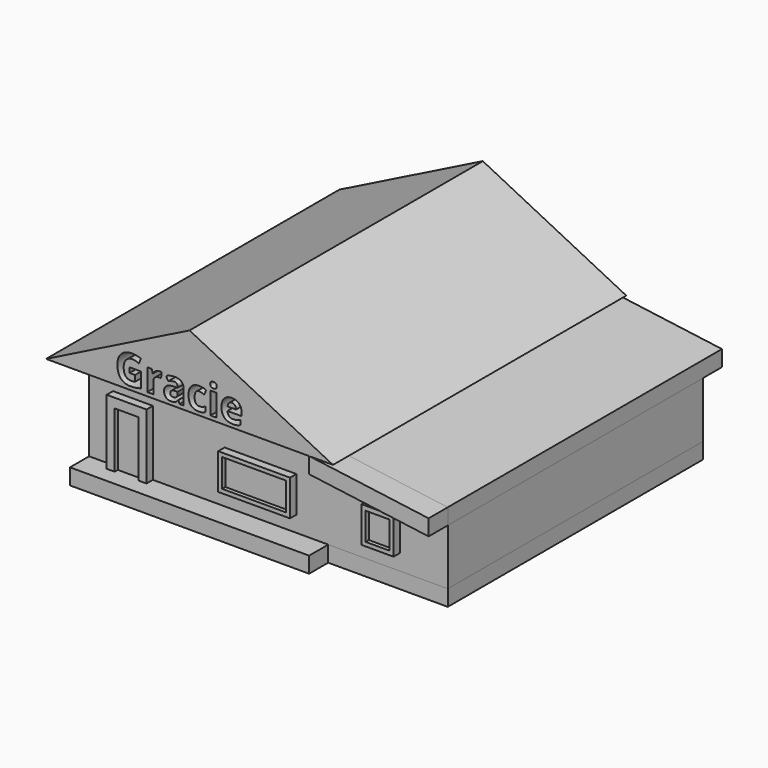
from build123d import *

# Parameters (mm, degrees)
F1_DEPTH      = 914.4
F2_DEPTH      = 13106.4
F3_DEPTH      = 12192
F4_DEPTH      = 914.4
F5_DEPTH      = 12192
F0_W          = 2743.2
F0_H          = 1371.6
F0_W_2        = 1219.2
F0_W_3        = 2438.4
F0_H_2        = 1071.7371232986
F0_W_4        = 914.4
F0_H_3        = 2133.6
F0_H_4        = 1049.4811702728
F6_DEPTH      = 12192
F7_DEPTH      = 304.8
F8_DEPTH      = 152.4
F0_W_5        = 4572
F0_H_5        = 609.6
F9_DEPTH      = 12192
F10_DEPTH     = 914.4
F11_DEPTH     = 13106.4
F12_TEXT_SIZE = 1537.0702371001
F13_DEPTH     = 1524


# Not quite as in the source:
# - Text() gives the source's letters only with a copy of the font that has no kerning and outlines rounded to 1/6400 em; it was checked with that copy


with BuildPart() as f1:
    # F0 (on Front) → F1 (new body)
    with BuildSketch(Plane.XZ):
        Polygon((0, 2286), (4572, 0), (5486.4, 0), (0, 2743.2), align=None)
        Polygon((-5486.4, 0), (-4572, 0), (0, 2286), (0, 2743.2), align=None)
    extrude(amount=F1_DEPTH)

    # F0 (on Front) → F2 (join)
    with BuildSketch(Plane.XZ):
        Polygon((-5486.4, 0), (-4572, 0), (0, 2286), (0, 2743.2), align=None)
        Polygon((0, 2286), (4572, 0), (5486.4, 0), (0, 2743.2), align=None)
    extrude(amount=-F2_DEPTH)

    # F0 (on Front) → F3 (join)
    with BuildSketch(Plane.XZ):
        Polygon((-4572, 0), (0, 0), (4572, 0), (0, 2286), align=None)
    extrude(amount=-F3_DEPTH)

    # F0 (on Front) → F4, piece 2 (join)
    with BuildSketch(Plane.XZ):
        Polygon((-4572, 0), (0, 0), (4572, 0), (0, 2286), align=None)
    extrude(amount=F4_DEPTH)

    # F12 (on Front) → F13 (cut)
    with BuildSketch(Plane.XZ):
        with Locations((-2848.2854366302, 141.368702054)):
            Text('Gracie', F12_TEXT_SIZE, font='Open Sans', font_style=FontStyle.BOLD, text_align=(TextAlign.LEFT, TextAlign.BOTTOM))
    extrude(amount=F13_DEPTH, mode=Mode.SUBTRACT)


with BuildPart() as f4:
    # F0 (on Front) → F4 (new body)
    with BuildSketch(Plane.XZ):
        Polygon((-3657.6, -3352.8), (-4572, -3352.8), (-4572, -3962.4), (4572, -3962.4), (4572, -3352.8), (-2133.6, -3352.8), (-2438.4, -3352.8), (-3352.8, -3352.8), align=None)
    extrude(amount=F4_DEPTH)

    # F0 (on Front) → F5 (join)
    with BuildSketch(Plane.XZ):
        Polygon((-3657.6, -3352.8), (-4572, -3352.8), (-4572, -3962.4), (4572, -3962.4), (4572, -3352.8), (-2133.6, -3352.8), (-2438.4, -3352.8), (-3352.8, -3352.8), align=None)
    extrude(amount=-F5_DEPTH)


with BuildPart() as f6:
    # F0 (on Front) → F6 (new body)
    with BuildSketch(Plane.XZ):
        Polygon((4572, 0), (0, 0), (-4572, 0), (-4572, -3352.8), (-3657.6, -3352.8), (-3657.6, -860.7614040375), (-2133.6, -860.7614040375), (-2133.6, -3352.8), (4572, -3352.8), (4572, -609.6), align=None)
        with Locations((1981.2, -2057.4)):
            Rectangle(F0_W, F0_H, mode=Mode.SUBTRACT)
        Polygon((9144, -1219.2), (4572, -609.6), (4572, -3352.8), (9144, -3352.8), align=None)
        with Locations((6705.6, -2058.8398735046)):
            Rectangle(F0_W_2, F0_H, mode=Mode.SUBTRACT)
        with Locations((1981.2, -2057.4)):
            Rectangle(F0_W, F0_H)
        with Locations((1981.2, -2054.9314383507)):
            Rectangle(F0_W_3, F0_H_2, mode=Mode.SUBTRACT)
        with Locations((1981.2, -2054.9314383507)):
            Rectangle(F0_W_3, F0_H_2)
        with Locations((-2895.6, -2286)):
            Rectangle(F0_W_4, F0_H_3)
        Polygon((-3657.6, -860.7614040375), (-3657.6, -3352.8), (-3352.8, -3352.8), (-3352.8, -1219.2), (-2438.4, -1219.2), (-2438.4, -3352.8), (-2133.6, -3352.8), (-2133.6, -860.7614040375), align=None)
        with Locations((6705.6, -2058.8398735046)):
            Rectangle(F0_W_2, F0_H)
        with Locations((6705.6, -2067.4992883682)):
            Rectangle(F0_W_4, F0_H_4, mode=Mode.SUBTRACT)
        with Locations((6705.6, -2067.4992883682)):
            Rectangle(F0_W_4, F0_H_4)
    extrude(amount=-F6_DEPTH)


with BuildPart() as f7:
    # F0 (on Front) → F7 (new body)
    with BuildSketch(Plane.XZ):
        Polygon((-3657.6, -860.7614040375), (-3657.6, -3352.8), (-3352.8, -3352.8), (-3352.8, -1219.2), (-2438.4, -1219.2), (-2438.4, -3352.8), (-2133.6, -3352.8), (-2133.6, -860.7614040375), align=None)
    extrude(amount=F7_DEPTH)


with BuildPart() as f7b:
    # F0 (on Front) → F7, piece 2 (new body)
    with BuildSketch(Plane.XZ):
        with Locations((1981.2, -2057.4)):
            Rectangle(F0_W, F0_H)
        with Locations((1981.2, -2054.9314383507)):
            Rectangle(F0_W_3, F0_H_2, mode=Mode.SUBTRACT)
    extrude(amount=F7_DEPTH)


with BuildPart() as f7c:
    # F0 (on Front) → F7, piece 3 (new body)
    with BuildSketch(Plane.XZ):
        with Locations((6705.6, -2058.8398735046)):
            Rectangle(F0_W_2, F0_H)
        with Locations((6705.6, -2067.4992883682)):
            Rectangle(F0_W_4, F0_H_4, mode=Mode.SUBTRACT)
    extrude(amount=F7_DEPTH)


with BuildPart() as f8:
    # F0 (on Front) → F8 (new body)
    with BuildSketch(Plane.XZ):
        with Locations((-2895.6, -2286)):
            Rectangle(F0_W_4, F0_H_3)
    extrude(amount=F8_DEPTH)


with BuildPart() as f8b:
    # F0 (on Front) → F8, piece 2 (new body)
    with BuildSketch(Plane.XZ):
        with Locations((1981.2, -2054.9314383507)):
            Rectangle(F0_W_3, F0_H_2)
    extrude(amount=F8_DEPTH)


with BuildPart() as f8c:
    # F0 (on Front) → F8, piece 3 (new body)
    with BuildSketch(Plane.XZ):
        with Locations((6705.6, -2067.4992883682)):
            Rectangle(F0_W_4, F0_H_4)
    extrude(amount=F8_DEPTH)


with BuildPart() as f9:
    # F0 (on Front) → F9 (new body)
    with BuildSketch(Plane.XZ):
        with Locations((6858, -3657.6)):
            Rectangle(F0_W_5, F0_H_5)
    extrude(amount=-F9_DEPTH)


with BuildPart() as f10:
    # F0 (on Front) → F10 (new body)
    with BuildSketch(Plane.XZ):
        Polygon((9144, -609.6), (4572, 0), (4572, -609.6), (9144, -1219.2), align=None)
    extrude(amount=F10_DEPTH)


with BuildPart() as f11:
    # F0 (on Front) → F11 (new body)
    with BuildSketch(Plane.XZ):
        Polygon((9144, -609.6), (4572, 0), (4572, -609.6), (9144, -1219.2), align=None)
    extrude(amount=-F11_DEPTH)


solid = Compound([f1.part, f4.part, f6.part, f7.part, f7b.part, f7c.part, f8.part, f8b.part, f8c.part, f9.part, f10.part, f11.part])
